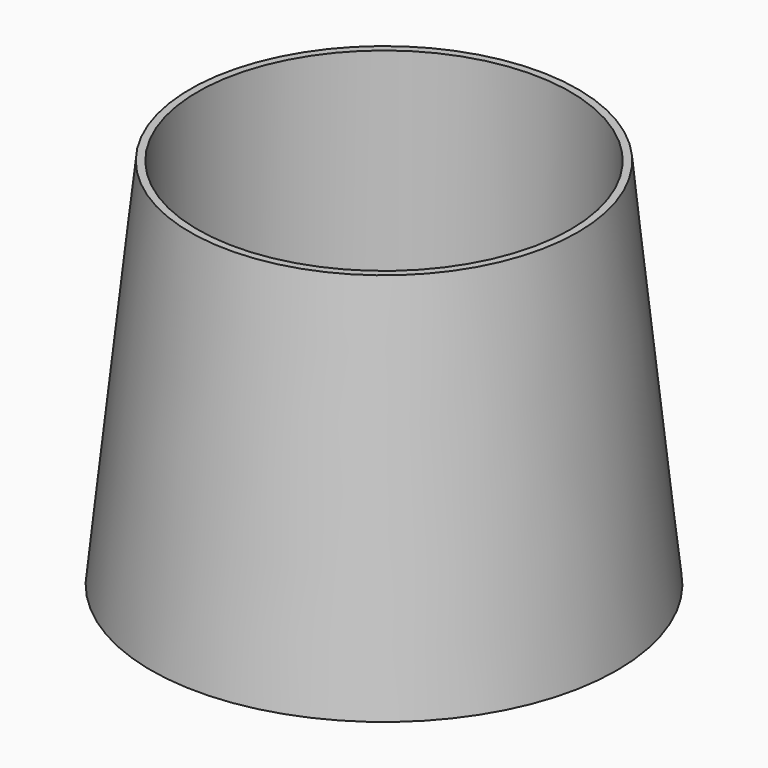
from build123d import *

# Parameters (mm, degrees)
F0_R     = 63.5
F0_R_2   = 50.8
F1_DEPTH = 101.6
F2_DEPTH = 12.7
F3_SIZE2 = 10.67858
F3_SIZE  = 101.59999


# Not quite as in the source:
# - a fillet or chamfer is up to 0.001 mm smaller than in the source, because OpenCascade refuses the exact size


with BuildPart() as f1:
    # F0 (on Top) → F1 (new body)
    with BuildSketch(Plane.XY):
        Circle(F0_R)
        Circle(F0_R_2, mode=Mode.SUBTRACT)
    extrude(amount=F1_DEPTH)

    # F0 (on Top) → F2 (join)
    with BuildSketch(Plane.XY):
        Circle(F0_R_2)
    extrude(amount=F2_DEPTH)

    # F3 (size 101.6 and 10.678590303 in the source; OpenCascade refuses exactly that, so slightly less here)
    f3_edges = [f1.edges().sort_by_distance(p)[0] for p in [
        (-63.5, 0, 101.6),
    ]]
    f3_side = f1.faces().sort_by_distance((-63.5, 0, 50.8))[0]
    chamfer(f3_edges, length=F3_SIZE, length2=F3_SIZE2, reference=f3_side)


solid = f1.part
